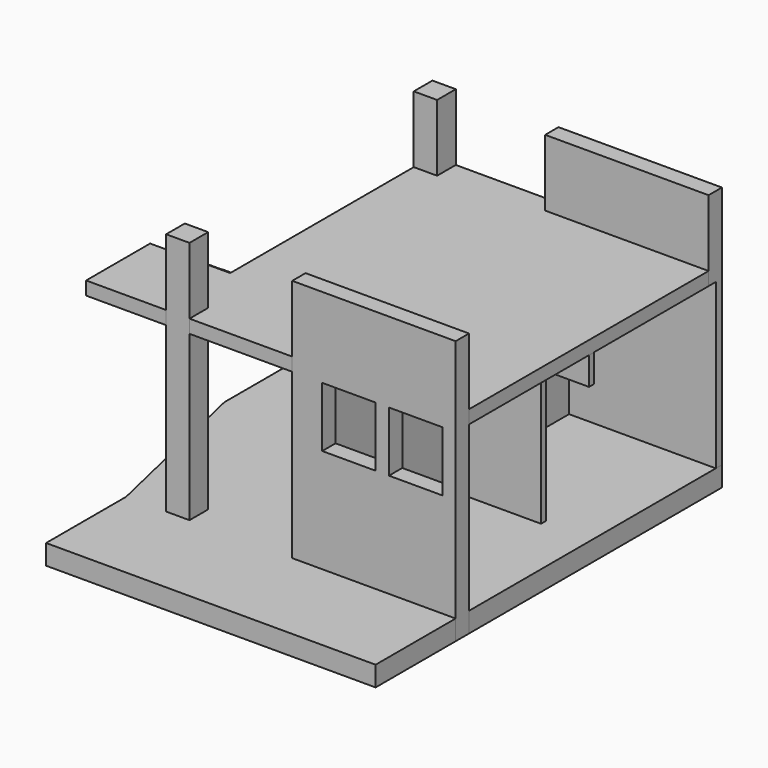
from build123d import *

# Parameters (mm, degrees)
F2_W          = 1480
F2_H          = 90
F2_W_2        = 350
F2_H_2        = 350
F2_W_3        = 250
F2_H_3        = 920
F2_H_4        = 135
F2_H_5        = 1230
F2_W_4        = 720
F3_DEPTH      = 300
F5_DEPTH      = 200
F6_DEPTH      = 2460
F7_START      = 2460
F7_DEPTH      = 1200
F8_DEPTH      = 3660
F8_DEPTH_BACK = 300
F9_W          = 271
F9_H          = 177
F10_DEPTH     = 1200
F11_DEPTH     = 2040
F12_W         = 800
F12_H         = 900
F13_DEPTH     = 250
F14_W         = 980
F14_H         = 1560
F15_DEPTH     = 250


# Not quite as in the source:
# - a feature names something its author has since deleted; it is built from what else it names


with BuildPart() as f3:
    # F2 (on Top) → F3 (new body)
    with BuildSketch(Plane.XY):
        Polygon((-4340, 4990), (-5540, 4990), (-5540, 2590), (-4940, 0), (-4340, 0), (-4340, 350), (-3990, 350), (-3990, 0), (-2450, 0), (-2450, 250), (-2450, 2590), (-2450, 3510), (-2450, 4740), (-2450, 4875), (-2450, 4990), (-3990, 4990), (-3990, 4640), (-4340, 4640), align=None)
        with Locations((-1460, 2545)):
            Rectangle(F2_W, F2_H)
        Polygon((-4340, 0), (-4940, 0), (-4940, -1500), (0, -1500), (0, 0), (-2450, 0), (-3990, 0), align=None)
        Polygon((0, 4990), (-2450, 4990), (-2450, 4875), (-2200, 4875), (-1229.6366691589, 4875), (0, 4875), align=None)
        with Locations((-4165, 4815)):
            Rectangle(F2_W_2, F2_H_2)
        with Locations((-4165, 175)):
            Rectangle(F2_W_2, F2_H_2)
        Polygon((-2200, 250), (0, 250), (0, 2500), (-720, 2500), (-2200, 2500), align=None)
        Polygon((-2450, 250), (-2450, 0), (0, 0), (0, 250), (-2200, 250), align=None)
        with Locations((-2325, 3050)):
            Rectangle(F2_W_3, F2_H_3)
        Polygon((0, 4740), (0, 4875), (-1229.6366691589, 4875), (-2200, 4875), (-2200, 4740), align=None)
        with Locations((-2325, 4807.5)):
            Rectangle(F2_W_3, F2_H_4)
        Polygon((-2450, 2590), (-2450, 250), (-2200, 250), (-2200, 2500), (-2200, 2590), align=None)
        with Locations((-2325, 4125)):
            Rectangle(F2_W_3, F2_H_5)
        Polygon((0, 2590), (0, 4740), (-2200, 4740), (-2200, 3510), (-2200, 2590), (-720, 2590), align=None)
        with Locations((-360, 2545)):
            Rectangle(F2_W_4, F2_H)
    extrude(amount=-F3_DEPTH)


with BuildPart() as f5:
    # F4 (on offset) → F5 (new body)
    with BuildSketch(Plane.XY.offset(2660)):
        Polygon((-4340, 1200), (-5540, 1200), (-5540, 0), (-4340, 0), (-4340, 175), (-3990, 175), (-3990, 0), (-2450, 0), (-2450, 175), (0, 175), (0, 4815), (-2450, 4815), (-2450, 4990), (-3990, 4990), (-3990, 4815), (-4165, 4815), (-4165, 4640), (-4340, 4640), align=None)
    extrude(amount=-F5_DEPTH)


with BuildPart() as f6:
    # F2 (on Top) → F6 (new body, through all)
    with BuildSketch(Plane.XY):
        Polygon((0, 4990), (-2450, 4990), (-2450, 4875), (-2200, 4875), (-1229.6366691589, 4875), (0, 4875), align=None)
        with Locations((-2325, 4807.5)):
            Rectangle(F2_W_3, F2_H_4)
        with Locations((-2325, 3050)):
            Rectangle(F2_W_3, F2_H_3)
        with Locations((-1460, 2545)):
            Rectangle(F2_W, F2_H)
        Polygon((-2450, 2590), (-2450, 250), (-2200, 250), (-2200, 2500), (-2200, 2590), align=None)
        with Locations((-2325, 4125)):
            Rectangle(F2_W_3, F2_H_5)
        with Locations((-360, 2545)):
            Rectangle(F2_W_4, F2_H)
    extrude(amount=F6_DEPTH)

    # F2 (on Top) → F7 (join)
    with BuildSketch(Plane.XY.offset(F7_START)):
        Polygon((0, 4740), (0, 4875), (-1229.6366691589, 4875), (-2200, 4875), (-2200, 4740), align=None)
        Polygon((0, 4990), (-2450, 4990), (-2450, 4875), (-2200, 4875), (-1229.6366691589, 4875), (0, 4875), align=None)
        with Locations((-2325, 4807.5)):
            Rectangle(F2_W_3, F2_H_4)
    extrude(amount=F7_DEPTH)

    # F2 (on Top) → F8 (join, two sides)
    with BuildSketch(Plane.XY) as f8_sk:
        Polygon((-2450, 250), (-2450, 0), (0, 0), (0, 250), (-2200, 250), align=None)
    extrude(amount=F8_DEPTH)
    extrude(f8_sk.sketch, amount=-F8_DEPTH_BACK)

    # F2 (on Top) → F11 (cut)
    with BuildSketch(Plane.XY):
        with Locations((-2325, 3050)):
            Rectangle(F2_W_3, F2_H_3)
        with Locations((-360, 2545)):
            Rectangle(F2_W_4, F2_H)
    extrude(amount=F11_DEPTH, mode=Mode.SUBTRACT)

    # F12 (on face) → F13 (cut, through all)
    with BuildSketch(Plane(origin=(0, 250, 0), x_dir=(-1, 0, 0), z_dir=(0, 1, 0))):
        with Locations((600, 2010)):
            Rectangle(F12_W, F12_H)
        with Locations((1600, 2010)):
            Rectangle(F12_W, F12_H)
    extrude(amount=-F13_DEPTH, mode=Mode.SUBTRACT)

    # F14 (on face) → F15 (cut, through all)
    with BuildSketch(Plane.YZ.offset(-2200)):
        with Locations((4250, 1680)):
            Rectangle(F14_W, F14_H)
    extrude(amount=-F15_DEPTH, mode=Mode.SUBTRACT)


with BuildPart() as f8:
    # F2 (on Top) → F8, piece 2 (new body, two sides)
    with BuildSketch(Plane.XY) as f8_2_sk:
        with Locations((-4165, 175)):
            Rectangle(F2_W_2, F2_H_2)
    extrude(amount=F8_DEPTH)
    extrude(f8_2_sk.sketch, amount=-F8_DEPTH_BACK)


with BuildPart() as f8b:
    # F2 (on Top) → F8, piece 3 (new body, two sides)
    with BuildSketch(Plane.XY) as f8_3_sk:
        with Locations((-4165, 4815)):
            Rectangle(F2_W_2, F2_H_2)
    extrude(amount=F8_DEPTH)
    extrude(f8_3_sk.sketch, amount=-F8_DEPTH_BACK)


with BuildPart() as f10:
    # F9 (on face) → F10 (new body)
    with BuildSketch(Plane(origin=(-4340, 0, 0), x_dir=(0, -1, 0), z_dir=(-1, 0, 0))):
        with Locations((-4854.5, 88.5)):
            Rectangle(F9_W, F9_H)
        Polygon((-4719, 177), (-4719, 0), (-4448, 177), align=None)
        with Locations((-4583.5, 265.5)):
            Rectangle(F9_W, F9_H)
        Polygon((-4448, 354), (-4448, 177), (-4177, 354), align=None)
        with Locations((-4312.5, 442.5)):
            Rectangle(F9_W, F9_H)
        Polygon((-4177, 531), (-4177, 354), (-3906, 531), align=None)
        with Locations((-4041.5, 619.5)):
            Rectangle(F9_W, F9_H)
        Polygon((-3906, 708), (-3906, 531), (-3635, 708), align=None)
        with Locations((-3770.5, 796.5)):
            Rectangle(F9_W, F9_H)
        Polygon((-3635, 885), (-3635, 708), (-3364, 885), align=None)
        with Locations((-3499.5, 973.5)):
            Rectangle(F9_W, F9_H)
        Polygon((-3364, 1062), (-3364, 885), (-3093, 1062), align=None)
        with Locations((-3228.5, 1150.5)):
            Rectangle(F9_W, F9_H)
        Polygon((-3093, 1239), (-3093, 1062), (-2822, 1239), align=None)
        with Locations((-2957.5, 1327.5)):
            Rectangle(F9_W, F9_H)
        Polygon((-2822, 1416), (-2822, 1239), (-2551, 1416), align=None)
        with Locations((-2686.5, 1504.5)):
            Rectangle(F9_W, F9_H)
        Polygon((-2551, 1593), (-2551, 1416), (-2280, 1593), align=None)
        with Locations((-2415.5, 1681.5)):
            Rectangle(F9_W, F9_H)
        Polygon((-2280, 1770), (-2280, 1593), (-2009, 1770), align=None)
        with Locations((-2144.5, 1858.5)):
            Rectangle(F9_W, F9_H)
        Polygon((-2009, 1947), (-2009, 1770), (-1738, 1947), align=None)
        with Locations((-1873.5, 2035.5)):
            Rectangle(F9_W, F9_H)
        Polygon((-1738, 2124), (-1738, 1947), (-1467, 2124), align=None)
        with Locations((-1602.5, 2212.5)):
            Rectangle(F9_W, F9_H)
        Polygon((-1467, 2301), (-1467, 2124), (-1196, 2301), align=None)
        with Locations((-1331.5, 2389.5)):
            Rectangle(F9_W, F9_H)
        Polygon((-1196, 2478), (-1196, 2301), (-925, 2478), align=None)
    extrude(amount=F10_DEPTH)


solid = Compound([f3.part, f5.part, f6.part, f8.part, f8b.part, f10.part])
